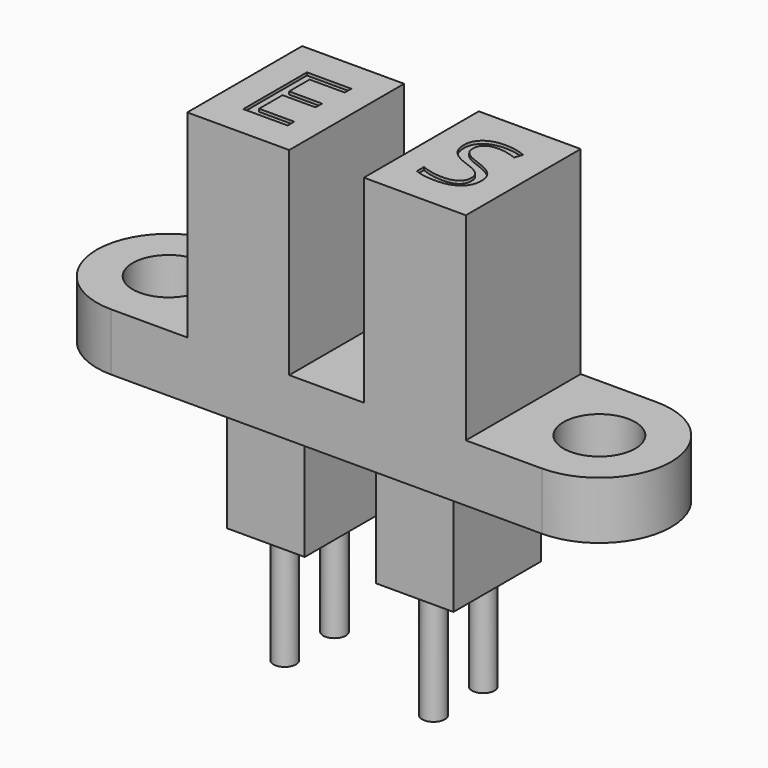
from build123d import *

# Parameters (mm, degrees)
F0_R           = 1.5875
F1_DEPTH       = 2.54
F2_W           = 4.5085
F2_H           = 6.35
F3_DEPTH       = 8.763
F4_TEXT_SIZE   = 4.9320618725
F4_TEXT_SIZE_2 = 4.8898376477
F5_DEPTH       = 0.125
F6_W           = 3.429
F6_H           = 4.826
F7_DEPTH       = 4.826
F8_R           = 0.5
F9_DEPTH       = 5


# Not quite as in the source:
# - Text() gives the source's letters only with a copy of the font that has no kerning and outlines rounded to 1/6400 em; it was checked with that copy


with BuildPart() as f1:
    # F0 (on Top) → F1 (new body)
    with BuildSketch(Plane.XY):
        with BuildLine():
            Line((-9.525, -3.175), (9.525, -3.175))
            ThreePointArc((9.525, -3.175), (12.7, 0), (9.525, 3.175))
            Line((9.525, 3.175), (-9.525, 3.175))
            ThreePointArc((-9.525, 3.175), (-12.7, 0), (-9.525, -3.175))
        make_face()
        with Locations((-9.525, 0)):
            Circle(F0_R, mode=Mode.SUBTRACT)
        with Locations((9.525, 0)):
            Circle(F0_R, mode=Mode.SUBTRACT)
    extrude(amount=F1_DEPTH)

    # F2 (on face) → F3 (join)
    with BuildSketch(Plane.XY.offset(2.54)):
        with Locations((-3.90525, 0)):
            Rectangle(F2_W, F2_H)
        with Locations((3.90525, 0)):
            Rectangle(F2_W, F2_H)
    extrude(amount=F3_DEPTH)

    # F4 (on face) → F5 (cut)
    with BuildSketch(Plane.XY.offset(11.303)):
        with Locations((-5.2885392283, -1.7755422741)):
            Text('E', F4_TEXT_SIZE, font='Open Sans', text_align=(TextAlign.LEFT, TextAlign.BOTTOM))
        with Locations((2.5219607717, -1.7603415532)):
            Text('S', F4_TEXT_SIZE_2, font='Open Sans', text_align=(TextAlign.LEFT, TextAlign.BOTTOM))
    extrude(amount=-F5_DEPTH, mode=Mode.SUBTRACT)

    # F6 (on face) → F7 (join)
    with BuildSketch(Plane.XY):
        with Locations((-3.2893, 0)):
            Rectangle(F6_W, F6_H)
        with Locations((3.2893, 0)):
            Rectangle(F6_W, F6_H)
    extrude(amount=-F7_DEPTH)

    # F8 (on face) → F9 (join)
    with BuildSketch(Plane(origin=(0, 0, -4.826), x_dir=(1, 0, 0), z_dir=(0, 0, -1))):
        with Locations((-3.2893, 1.375)):
            Circle(F8_R)
        with Locations((-3.2893, -1.375)):
            Circle(F8_R)
        with Locations((3.2893, 1.375)):
            Circle(F8_R)
        with Locations((3.2893, -1.375)):
            Circle(F8_R)
    extrude(amount=F9_DEPTH)


solid = f1.part
